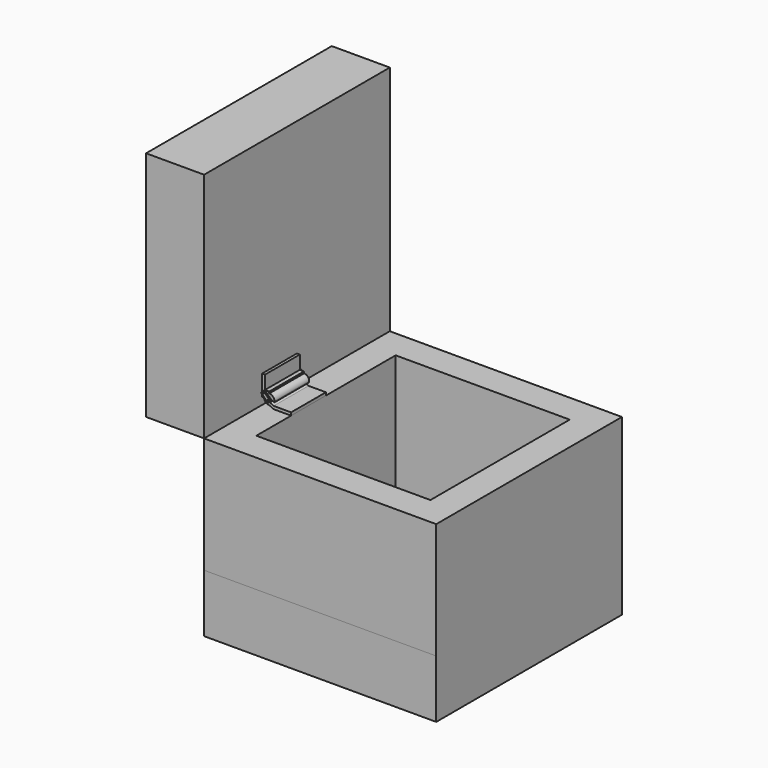
from build123d import *

# Parameters (mm, degrees)
F0_W      = 50.8
F0_H      = 50.8
F0_W_2    = 38.1
F0_H_2    = 38.1
F1_DEPTH  = 25.4
F2_W      = 50.8
F2_H      = 50.8
F3_DEPTH  = 12.7
F4_W      = 50.8
F4_H      = 12.7
F5_DEPTH  = 50.8
F6_ANGLE  = 90
F7_W      = 3.81
F7_H      = 0.635
F8_DEPTH  = 9.525
F10_DEPTH = 9.525
F11_DEPTH = 9.525
F9_R      = 0.5077030433
F12_DEPTH = 9.525
F13_R     = 0.127
F15_DEPTH = 0.381
F14_R     = 0.127
F16_DEPTH = 0.381
F17_DEPTH = 0.762
F18_DEPTH = 0.762


# Not quite as in the source:
# - a feature names something its author has since deleted; it is built from what else it names


with BuildPart() as f1:
    # F0 (on Top) → F1 (new body)
    with BuildSketch(Plane.XY):
        with Locations((25.4, 0.0146500111)):
            Rectangle(F0_W, F0_H)
        with Locations((25.4, 0.0146500111)):
            Rectangle(F0_W_2, F0_H_2, mode=Mode.SUBTRACT)
    extrude(amount=F1_DEPTH)

    # F2 (on Top) → F3 (join)
    with BuildSketch(Plane.XY):
        with Locations((25.4, 0.0146146208)):
            Rectangle(F2_W, F2_H)
    extrude(amount=-F3_DEPTH)


with BuildPart() as f5:
    # F4 (on Right) → F5 (new body)
    with BuildSketch(Plane.YZ):
        with Locations((0.0146406978, 31.7500369459)):
            Rectangle(F4_W, F4_H)
    extrude(amount=F5_DEPTH)


with BuildPart() as f5_1:
    # F6: moved
    add(f5.part.rotate(Axis((0, 0.0146406978, 25.4000369459), (0, -1, 0)), F6_ANGLE))


with BuildPart() as f8:
    # F7 (on Front) → F8 (new body)
    with BuildSketch(Plane.XZ):
        with Locations((4.4450491789, 25.7175220448)):
            Rectangle(F7_W, F7_H)
    extrude(amount=F8_DEPTH)

    # F7 (on Front) → F10 (join)
    with BuildSketch(Plane.XZ):
        with Locations((4.4450491789, 25.7175220448)):
            Rectangle(F7_W, F7_H)
        with BuildLine():
            Line((2.5400491789, 25.4000220448), (2.5400491789, 26.0350220448))
            Line((2.5400491789, 26.0350220448), (1.5873330849, 26.4795220448))
            ThreePointArc((1.5873330849, 26.4795220448), (1.1684398268, 27.3027162398), (2.0661893734, 27.085538902))
            Line((2.0661893734, 27.085538902), (2.0874672369, 26.9772455298))
            Line((2.0874672369, 26.9772455298), (2.7012227073, 26.7624311151))
            Line((2.7012227073, 26.7624311151), (2.7011893485, 26.9876899582))
            ThreePointArc((2.7011893485, 26.9876899582), (0.7677044508, 27.7914004341), (1.5611574045, 25.8536835329))
            Line((1.5611574045, 25.8536835329), (2.5400491789, 25.4000220448))
        make_face()
    extrude(amount=F10_DEPTH)


with BuildPart() as f11:
    # F9 (on Front) → F11 (new body)
    with BuildSketch(Plane.XZ):
        with BuildLine():
            Line((0, 31.4426555759), (0, 28.2714386624))
            Line((0, 28.2714386624), (0, 27.6326555759))
            Line((0, 27.6326555759), (0, 26.9874893129))
            Line((0, 26.9874893129), (0.4331566452, 26.9874893129))
            ThreePointArc((0.4331566452, 26.9874893129), (0.4848538675, 27.3254725509), (0.635, 27.6326555759))
            ThreePointArc((0.635, 27.6326555759), (1.041532233, 27.9908455658), (1.5673746821, 28.1214527786))
            Line((1.5673746821, 28.1214527786), (1.5673746821, 28.499443084))
            Line((1.5673746821, 28.499443084), (0.635, 28.499443084))
            Line((0.635, 28.499443084), (0.635, 31.4426555759))
            Line((0.635, 31.4426555759), (0, 31.4426555759))
        make_face()
    extrude(amount=F11_DEPTH)


with BuildPart() as f12:
    # F9 (on Front) → F12 (new body)
    with BuildSketch(Plane.XZ):
        with Locations((1.5672598965, 26.9874893129)):
            Circle(F9_R)
    extrude(amount=F12_DEPTH)


with BuildPart() as f15:
    # F13 (on face) → F15 (new body)
    with BuildSketch(Plane.XZ):
        Polygon((0.0522972679, 27.9557561948), (1.0593642086, 26.9875489975), (1.5873443298, 26.4799420722), (2.0753642007, 26.9875489975), (1.5673642047, 27.4955489935), (0.560297264, 28.4637561908), align=None)
        with Locations((1.5673642047, 26.9874855876)):
            Circle(F13_R, mode=Mode.SUBTRACT)
        with Locations((0.567795408, 27.9552003249)):
            Circle(F13_R, mode=Mode.SUBTRACT)
    extrude(amount=-F15_DEPTH)


with BuildPart() as f16:
    # F14 (on face) → F16 (new body)
    with BuildSketch(Plane.XZ.offset(9.525)):
        Polygon((0.052330317, 27.9558002949), (1.0593972577, 26.9875930976), (1.5873773788, 26.4799861723), (2.0753972498, 26.9875930976), (1.5673972537, 27.4955930936), (0.560330313, 28.4638002909), align=None)
        with Locations((1.5673972537, 26.9875296877)):
            Circle(F14_R, mode=Mode.SUBTRACT)
        with Locations((0.5429185112, 27.9876943678)):
            Circle(F14_R, mode=Mode.SUBTRACT)
    extrude(amount=F16_DEPTH)


with BuildPart() as f17_tool:
    # F13 (on face) → F17 (new body)
    with BuildSketch(Plane.XZ):
        with Locations((1.5673642047, 26.9874855876)):
            Circle(F13_R)
        with Locations((0.567795408, 27.9552003249)):
            Circle(F13_R)
    extrude(amount=F17_DEPTH)


with BuildPart() as f11_1:
    add(f11.part)

    # F17: cut by f17_tool
    add(f17_tool.part, mode=Mode.SUBTRACT)


with BuildPart() as f12_1:
    add(f12.part)

    # F17: cut by f17_tool
    add(f17_tool.part, mode=Mode.SUBTRACT)


with BuildPart() as f18_tool:
    # F14 (on face) → F18 (new body)
    with BuildSketch(Plane.XZ.offset(9.525)):
        with Locations((1.5673972537, 26.9875296877)):
            Circle(F14_R)
        with Locations((0.5429185112, 27.9876943678)):
            Circle(F14_R)
    extrude(amount=-F18_DEPTH)


with BuildPart() as f11_2:
    add(f11_1.part)

    # F18: cut by f18_tool
    add(f18_tool.part, mode=Mode.SUBTRACT)


with BuildPart() as f12_2:
    add(f12_1.part)

    # F18: cut by f18_tool
    add(f18_tool.part, mode=Mode.SUBTRACT)


solid = Compound([f1.part, f5_1.part, f8.part, f15.part, f16.part, f11_2.part, f12_2.part])
